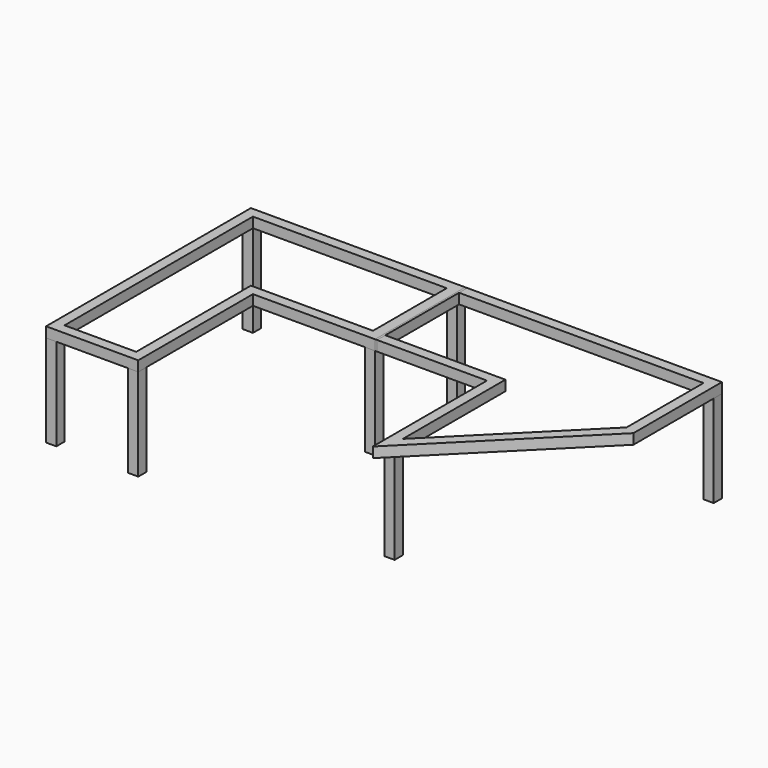
from build123d import *

# Parameters (mm, degrees)
F1_DEPTH = 50
F2_DEPTH = 50
F3_DEPTH = 50
F4_T     = -2
F5_W     = 50
F5_H     = 50
F6_DEPTH = 450
F7_T     = -2


# Not quite as in the source:
# - a shell that OpenCascade refuses in one call is made with other operations: the cavity is built on its own and cut out


with BuildPart() as f1:
    # F0 (on Top) → F1 (new body)
    with BuildSketch(Plane.XY):
        Polygon((1278.5535, 275), (35, 275), (35, 225), (1228.5535, 225), align=None)
        Polygon((35, -225), (35, -275), (571.4467188135, -275), (621.4467188135, -225), align=None)
        Polygon((1278.5535, -265), (1278.5535, 275), (1228.5535, 225), (1228.5535, -244.2893218813), align=None)
        Polygon((621.4467188135, -851.3961030679), (571.4467188135, -901.3961030679), (571.4467188135, -972.1067811865), (1278.5535, -265), (1228.5535, -244.2893218813), align=None)
        Polygon((621.4467188135, -225), (571.4467188135, -275), (571.4467188135, -901.3961030679), (621.4467188135, -851.3961030679), align=None)
    extrude(amount=-F1_DEPTH)

    # F4#2 (hollow: no face is removed)
    offset(amount=F4_T, kind=Kind.INTERSECTION, mode=Mode.SUBTRACT)


with BuildPart() as f2:
    # F0 (on Top) → F2 (new body)
    with BuildSketch(Plane.XY):
        Polygon((-1021.4465, 275), (-1021.4465, -975), (-971.4465, -925), (-971.4465, 225), align=None)
        Polygon((-1021.4465, -975), (-571.4465, -975), (-621.4465, -925), (-971.4465, -925), align=None)
        Polygon((-621.4465, -925), (-571.4465, -975), (-571.4465, -275), (-621.4465, -225), align=None)
        Polygon((25, 275), (-1021.4465, 275), (-971.4465, 225), (-25, 225), align=None)
        Polygon((-621.4465, -225), (-571.4465, -275), (25, -275), (-25, -225), align=None)
        Polygon((-25, -225), (25, -275), (25, 275), (-25, 225), align=None)
    extrude(amount=-F2_DEPTH)

    # F4 (hollow: no face is removed)
    offset(amount=F4_T, kind=Kind.INTERSECTION, mode=Mode.SUBTRACT)


with BuildPart() as f3:
    # F0 (on Top) → F3 (new body)
    with BuildSketch(Plane.XY):
        Polygon((25, 275), (25, -275), (35, -275), (35, -225), (35, 225), (35, 275), align=None)
    extrude(amount=-F3_DEPTH)


with BuildPart() as f6:
    # F5 (on face) → F6 (new body)
    with BuildSketch(Plane(origin=(0, 0, -50), x_dir=(1, 0, 0), z_dir=(0, 0, -1))):
        with Locations((-996.4465, 950)):
            Rectangle(F5_W, F5_H)
        with Locations((-996.4465, -250)):
            Rectangle(F5_W, F5_H)
        with Locations((1253.5535, -250)):
            Rectangle(F5_W, F5_H)
        with Locations((596.4467188135, 876.3961030679)):
            Rectangle(F5_W, F5_H)
        with Locations((-596.4465, 950)):
            Rectangle(F5_W, F5_H)
        with Locations((0, 250)):
            Rectangle(F5_W, F5_H)
        with Locations((0, -250)):
            Rectangle(F5_W, F5_H)
    extrude(amount=F6_DEPTH)

    # F7: a shell. OpenCascade refuses it in one call, so the cavity is built on its own and cut out:
    # the body offset inwards by the wall thickness, plus a prism from it out through each open face.
    f7_core = offset(f6.part, amount=F7_T, mode=Mode.PRIVATE)
    f7_exits = [f7_core.faces().sort_by_distance(p)[0] for p in [
        (-996.4465, 250, -52),
        (-996.4465, -950, -52),
        (-996.4465, -950, -498),
        (-996.4465, 250, -498),
        (596.446719, -876.396103, -498),
        (1253.5535, 250, -498),
        (596.446719, -876.396103, -52),
        (1253.5535, 250, -52),
        (-596.4465, -950, -498),
        (-596.4465, -950, -52),
        (0, -250, -498),
        (0, 250, -498),
    ]]
    add(f7_core, mode=Mode.SUBTRACT)
    extrude(f7_exits, amount=-F7_T, mode=Mode.SUBTRACT)


solid = Compound([f1.part, f2.part, f3.part, f6.part])
